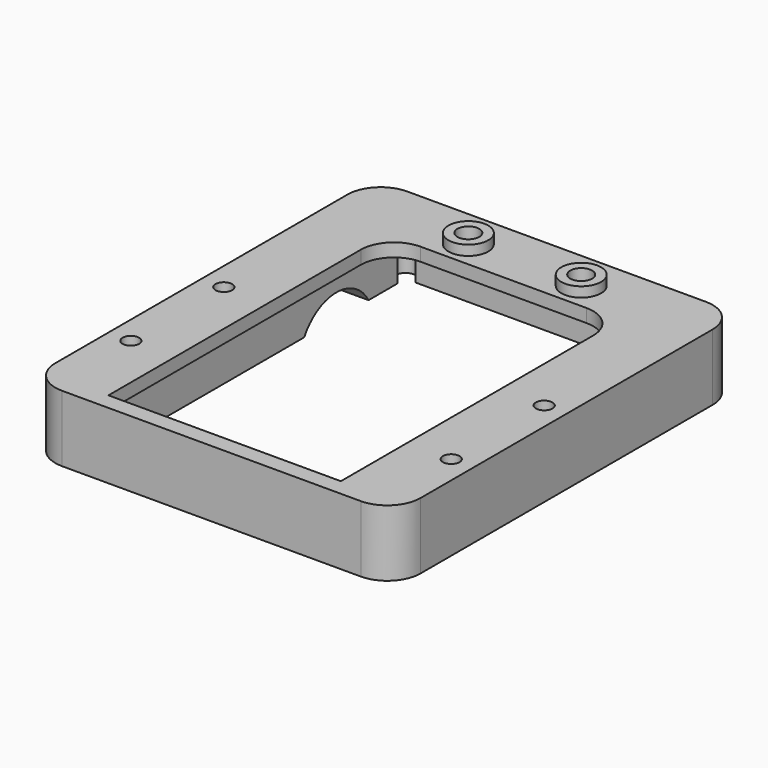
from build123d import *

# Parameters (mm, degrees)
F0_W            = 55
F0_H            = 10
F1_DEPTH        = 32.5
F3_R            = 5
F4_DEPTH        = 12.5
F6_DEPTH        = 30
F7_DEPTH        = 3
F9_D            = 3.3
F9_CSINK_D      = 6.72
F9_CSINK_ANGLE  = 90
F10_R           = 3
F11_DEPTH       = 1.5
F12_D           = 3.3
F12_DEPTH       = 13.5
F12_CSINK_D     = 6.72
F12_CSINK_ANGLE = 90
F12_TIP         = 0.9914200214
F14_D           = 2.5
F14_DEPTH       = 13.5
F14_TIP         = 0.7510757738
F16_DEPTH       = 12


# Not quite as in the source:
# - a feature names something its author has since deleted; it is built from what else it names


with BuildPart() as f1:
    # F0 (on Front) → F1 (new body, symmetric)
    with BuildSketch(Plane.XZ):
        Rectangle(F0_W, F0_H)
    extrude(amount=F1_DEPTH, both=True)

    # F3
    f3_edges = [f1.edges().sort_by_distance(p)[0] for p in [
        (27.5, -32.5, 0),
        (-27.5, -32.5, 0),
        (-27.5, 32.5, 0),
        (27.5, 32.5, 0),
    ]]
    fillet(f3_edges, radius=F3_R)

    # F2 (on Top) → F4 (cut, symmetric)
    with BuildSketch(Plane.XY):
        with BuildLine():
            ThreePointArc((-12.5, 22.5), (-16.0355339059, 21.0355339059), (-17.5, 17.5))
            Line((-17.5, 17.5), (-17.5, -30))
            Line((-17.5, -30), (17.5, -30))
            Line((17.5, -30), (17.5, 17.5))
            ThreePointArc((17.5, 17.5), (16.0355339059, 21.0355339059), (12.5, 22.5))
            Line((12.5, 22.5), (-12.5, 22.5))
        make_face()
    extrude(amount=F4_DEPTH, both=True, mode=Mode.SUBTRACT)

    # F5 (on Top) → F6 (cut)
    with BuildSketch(Plane.XY):
        with BuildLine():
            ThreePointArc((-20.75, -28.5), (-21.8106601718, -31.0606601718), (-19.25, -30))
            Line((-19.25, -30), (-20.75, -30))
            Line((-20.75, -30), (-20.75, -28.5))
        make_face()
        with BuildLine():
            ThreePointArc((-20.75, -28.5), (-19.6893398282, -28.9393398282), (-19.25, -30))
            Line((-19.25, -30), (19.25, -30))
            ThreePointArc((19.25, -30), (19.6893398282, -28.9393398282), (20.75, -28.5))
            Line((20.75, -28.5), (20.75, 28.5))
            ThreePointArc((20.75, 28.5), (19.6893398282, 28.9393398282), (19.25, 30))
            Line((19.25, 30), (-19.25, 30))
            ThreePointArc((-19.25, 30), (-19.6893398282, 28.9393398282), (-20.75, 28.5))
            Line((-20.75, 28.5), (-20.75, -28.5))
        make_face()
        with BuildLine():
            Line((-20.75, -30), (-19.25, -30))
            ThreePointArc((-19.25, -30), (-19.6893398282, -28.9393398282), (-20.75, -28.5))
            Line((-20.75, -28.5), (-20.75, -30))
        make_face()
        with BuildLine():
            ThreePointArc((20.75, -28.5), (19.6893398282, -28.9393398282), (19.25, -30))
            Line((19.25, -30), (20.75, -30))
            Line((20.75, -30), (20.75, -28.5))
        make_face()
        with BuildLine():
            Line((20.75, -30), (19.25, -30))
            ThreePointArc((19.25, -30), (20.75, -31.5), (22.25, -30))
            ThreePointArc((22.25, -30), (21.8106601718, -28.9393398282), (20.75, -28.5))
            Line((20.75, -28.5), (20.75, -30))
        make_face()
        with BuildLine():
            ThreePointArc((-19.25, 30), (-21.8106601718, 31.0606601718), (-20.75, 28.5))
            Line((-20.75, 28.5), (-20.75, 30))
            Line((-20.75, 30), (-19.25, 30))
        make_face()
        with BuildLine():
            Line((-20.75, 30), (-20.75, 28.5))
            ThreePointArc((-20.75, 28.5), (-19.6893398282, 28.9393398282), (-19.25, 30))
            Line((-19.25, 30), (-20.75, 30))
        make_face()
        with BuildLine():
            ThreePointArc((19.25, 30), (19.6893398282, 28.9393398282), (20.75, 28.5))
            Line((20.75, 28.5), (20.75, 30))
            Line((20.75, 30), (19.25, 30))
        make_face()
        with BuildLine():
            Line((20.75, 30), (20.75, 28.5))
            ThreePointArc((20.75, 28.5), (21.8106601718, 28.9393398282), (22.25, 30))
            ThreePointArc((22.25, 30), (20.75, 31.5), (19.25, 30))
            Line((19.25, 30), (20.75, 30))
        make_face()
    extrude(amount=-F6_DEPTH, mode=Mode.SUBTRACT)

    # F5 (on Top) → F7 (cut)
    with BuildSketch(Plane.XY):
        with BuildLine():
            ThreePointArc((-20.75, -28.5), (-21.8106601718, -31.0606601718), (-19.25, -30))
            Line((-19.25, -30), (-20.75, -30))
            Line((-20.75, -30), (-20.75, -28.5))
        make_face()
        with BuildLine():
            ThreePointArc((-20.75, -28.5), (-19.6893398282, -28.9393398282), (-19.25, -30))
            Line((-19.25, -30), (19.25, -30))
            ThreePointArc((19.25, -30), (19.6893398282, -28.9393398282), (20.75, -28.5))
            Line((20.75, -28.5), (20.75, 28.5))
            ThreePointArc((20.75, 28.5), (19.6893398282, 28.9393398282), (19.25, 30))
            Line((19.25, 30), (-19.25, 30))
            ThreePointArc((-19.25, 30), (-19.6893398282, 28.9393398282), (-20.75, 28.5))
            Line((-20.75, 28.5), (-20.75, -28.5))
        make_face()
        with BuildLine():
            Line((-20.75, -30), (-19.25, -30))
            ThreePointArc((-19.25, -30), (-19.6893398282, -28.9393398282), (-20.75, -28.5))
            Line((-20.75, -28.5), (-20.75, -30))
        make_face()
        with BuildLine():
            ThreePointArc((20.75, -28.5), (19.6893398282, -28.9393398282), (19.25, -30))
            Line((19.25, -30), (20.75, -30))
            Line((20.75, -30), (20.75, -28.5))
        make_face()
        with BuildLine():
            Line((20.75, -30), (19.25, -30))
            ThreePointArc((19.25, -30), (20.75, -31.5), (22.25, -30))
            ThreePointArc((22.25, -30), (21.8106601718, -28.9393398282), (20.75, -28.5))
            Line((20.75, -28.5), (20.75, -30))
        make_face()
        with BuildLine():
            ThreePointArc((-19.25, 30), (-21.8106601718, 31.0606601718), (-20.75, 28.5))
            Line((-20.75, 28.5), (-20.75, 30))
            Line((-20.75, 30), (-19.25, 30))
        make_face()
        with BuildLine():
            Line((-20.75, 30), (-20.75, 28.5))
            ThreePointArc((-20.75, 28.5), (-19.6893398282, 28.9393398282), (-19.25, 30))
            Line((-19.25, 30), (-20.75, 30))
        make_face()
        with BuildLine():
            ThreePointArc((19.25, 30), (19.6893398282, 28.9393398282), (20.75, 28.5))
            Line((20.75, 28.5), (20.75, 30))
            Line((20.75, 30), (19.25, 30))
        make_face()
        with BuildLine():
            Line((20.75, 30), (20.75, 28.5))
            ThreePointArc((20.75, 28.5), (21.8106601718, 28.9393398282), (22.25, 30))
            ThreePointArc((22.25, 30), (20.75, 31.5), (19.25, 30))
            Line((19.25, 30), (20.75, 30))
        make_face()
    extrude(amount=F7_DEPTH, mode=Mode.SUBTRACT)

    # F9 (through all)
    with Locations(Plane(origin=(0, 0, 3), x_dir=(1, 0, 0), z_dir=(0, 0, -1))):
        with Locations((-8.5, -26.5042820722), (8.5, -26.5042820722)):
            CounterSinkHole(F9_D / 2, F9_CSINK_D / 2, counter_sink_angle=F9_CSINK_ANGLE)

    # F10 (on face) → F11 (join)
    with BuildSketch(Plane.XY.offset(5)):
        with Locations((8.5, 26.5042820722)):
            Circle(F10_R)
        with Locations((-8.5, 26.5042820722)):
            Circle(F10_R)
    extrude(amount=F11_DEPTH)

    # F12
    with Locations(Plane(origin=(0, 0, 3), x_dir=(1, 0, 0), z_dir=(0, 0, -1))):
        with Locations((-8.5, -26.5042820722), (8.5, -26.5042820722)):
            CounterSinkHole(F12_D / 2, F12_CSINK_D / 2, depth=F12_DEPTH, counter_sink_angle=F12_CSINK_ANGLE)
            with Locations((0, 0, -(F12_DEPTH + F12_TIP / 2))):  # 118° drill point
                Cone(0, F12_D / 2, F12_TIP, mode=Mode.SUBTRACT)

    # F14
    with Locations(Plane(origin=(0, 0, -5), x_dir=(1, 0, 0), z_dir=(0, 0, -1))):
        with Locations((-24.125, 0), (24.125, 0), (-24.125, 17.5), (24.125, 17.5)):
            Hole(F14_D / 2, depth=F14_DEPTH)
            with Locations((0, 0, -(F14_DEPTH + F14_TIP / 2))):  # 118° drill point
                Cone(0, F14_D / 2, F14_TIP, mode=Mode.SUBTRACT)

    # F15 (on face) → F16 (cut)
    with BuildSketch(Plane(origin=(-27.5, 0, 0), x_dir=(0, -1, 0), z_dir=(-1, 0, 0))):
        with BuildLine():
            Line((-23.0304132, -5), (-10.906057547, -5))
            ThreePointArc((-10.906057547, -5), (-16.9682353735, -1.5), (-23.0304132, -5))
        make_face()
    extrude(amount=-F16_DEPTH, mode=Mode.SUBTRACT)


solid = f1.part
